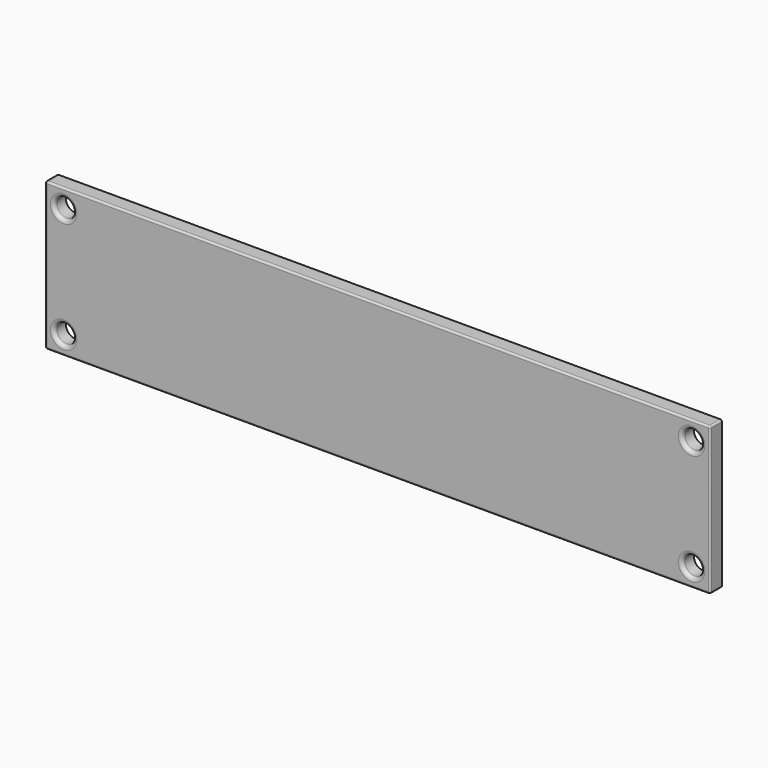
from build123d import *

# Parameters (mm, degrees)
F0_W         = 180
F0_H         = 40
F0_R         = 2.5751263091
F1_DEPTH     = 4
F2_R         = 1
F3_R         = 0.5
F4_TEXT_SIZE = 8.1141045959
F5_DEPTH     = 1


# Not quite as in the source:
# - a feature names something its author has since deleted; it is built from what else it names
# - Text() gives the source's letters only with a copy of the font that has no kerning and outlines rounded to 1/6400 em; it was checked with that copy


with BuildPart() as f1:
    # F0 (on Front) → F1 (new body)
    with BuildSketch(Plane.XZ):
        Rectangle(F0_W, F0_H)
        with Locations((-85, -15)):
            Circle(F0_R, mode=Mode.SUBTRACT)
        with Locations((85, -15)):
            Circle(F0_R, mode=Mode.SUBTRACT)
        with Locations((-85, 15)):
            Circle(F0_R, mode=Mode.SUBTRACT)
        with Locations((85, 15)):
            Circle(F0_R, mode=Mode.SUBTRACT)
    extrude(amount=F1_DEPTH)

    # F2
    f2_edges = [f1.edges().sort_by_distance(p)[0] for p in [
        (-87.575126, -4, 15),
        (-87.575126, -4, -15),
        (82.424874, -4, 15),
        (82.424874, -4, -15),
    ]]
    fillet(f2_edges, radius=F2_R)

    # F3
    f3_edges = [f1.edges().sort_by_distance(p)[0] for p in [
        (0, -4, 20),
        (-90, -4, 0),
        (0, -4, -20),
        (90, -4, 0),
        (-90, -2, 20),
        (-90, -2, -20),
        (90, -2, 20),
        (90, -2, -20),
    ]]
    fillet(f3_edges, radius=F3_R)

    # F4 (on face) → F5 (join)
    with BuildSketch(Plane(origin=(0, 0, 0), x_dir=(-1, 0, 0), z_dir=(0, 1, 0))):
        with Locations((-70.5961091444, -3.0954065128)):
            Text('Berea Cigar Cap', F4_TEXT_SIZE, font='Open Sans', text_align=(TextAlign.LEFT, TextAlign.BOTTOM))
    extrude(amount=F5_DEPTH)

    # F6: F1 across plane


with BuildPart() as f1_1:
    add(f1.part)
    add(f1.part.mirror(Plane.YZ))


solid = f1_1.part
